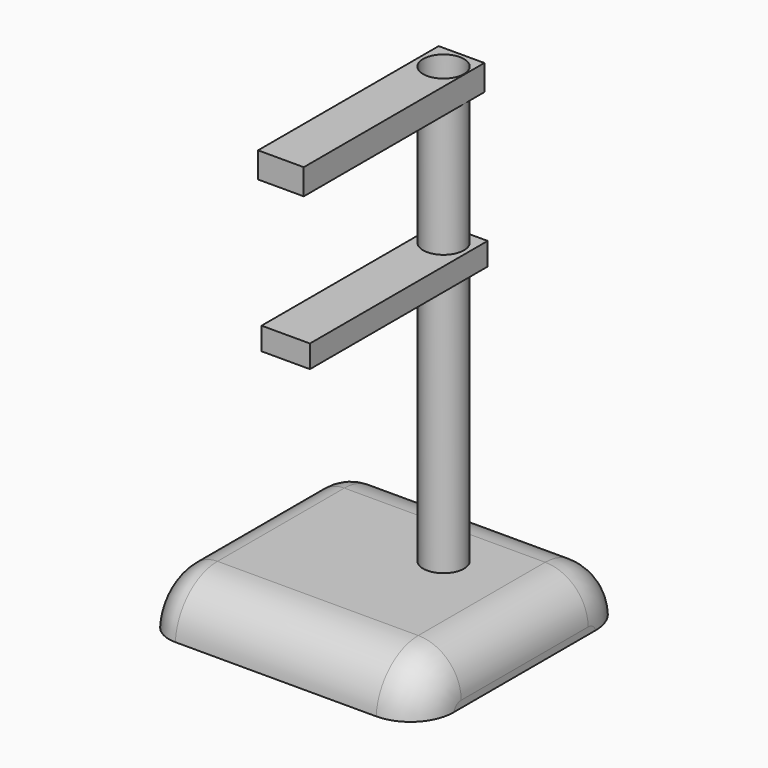
from build123d import *

# Parameters (mm, degrees)
F0_W        = 93.7904641032
F0_H        = 89.8338183761
F1_DEPTH    = 16.9549565762
F2_T1_DEPTH = 183.3558146052
F3_R        = 10.7925712466
F4_R        = 14.6181693704
F5_R        = 6.9569907431
F6_DEPTH    = 112.9271313548
F8_W        = 16.4551511407
F8_H        = 75.6539739668
F9_DEPTH    = 7.6955053955
F10_DEPTH   = 43.5431748629
F11_W       = 15.558283776
F11_H       = 76.8622979522
F11_R       = 6.9569907431
F12_DEPTH   = 8.7455324829


# Not quite as in the source:
# - a fillet or chamfer that OpenCascade refuses, or shapes differently, is made with other operations: its cross-section is extruded or revolved along the edge and cut away or added


with BuildPart() as f1:
    # F0 (on Top) → F1 (new body)
    with BuildSketch(Plane.XY):
        with Locations((8.7873749435, 5.4381676018)):
            Rectangle(F0_W, F0_H)
    extrude(amount=F1_DEPTH)

    # F2: fillet of radius 17.9401412852 on 2 edges, made by hand

    # F2_s2 → F2_t1 (cut)
    with BuildSketch(Plane.YZ.offset(-82.8905323591)):
        with BuildLine():
            ThreePointArc((-39.4787415862, 0), (-33.8980337182, 12.0440712599), (-21.5656714858, 16.9549565762))
            Line((-21.5656714858, 16.9549565762), (-39.4787415862, 16.9549565762))
            Line((-39.4787415862, 16.9549565762), (-39.4787415862, 0))
        make_face()
        with BuildLine():
            ThreePointArc((50.3550767899, 0), (44.7743689219, 12.0440712599), (32.4420066895, 16.9549565762))
            Line((32.4420066895, 16.9549565762), (50.3550767899, 16.9549565762))
            Line((50.3550767899, 16.9549565762), (50.3550767899, 0))
        make_face()
    extrude(amount=F2_T1_DEPTH, mode=Mode.SUBTRACT)

    # F3
    f3_edges = [f1.edges().sort_by_distance(p)[0] for p in [
        (-38.107857, 5.438168, 16.954957),
        (-38.107857, -33.898034, 12.044071),
        (-38.107857, 44.774369, 12.044071),
    ]]
    fillet(f3_edges, radius=F3_R)

    # F4
    f4_edges = [f1.edges().sort_by_distance(p)[0] for p in [
        (55.682607, 44.774369, 12.044071),
        (55.682607, 5.438168, 16.954957),
        (55.682607, -33.898034, 12.044071),
    ]]
    fillet(f4_edges, radius=F4_R)

    # F5 (on Top) → F6 (join)
    with BuildSketch(Plane.XY):
        with Locations((19.552404061, 16.0813909024)):
            Circle(F5_R)
    extrude(amount=F6_DEPTH)

    # F8 (on offset) → F9 (join)
    with BuildSketch(Plane.XY.offset(112.385711167)):
        with Locations((19.8183581233, -13.5854128748)):
            Rectangle(F8_W, F8_H)
    extrude(amount=-F9_DEPTH)

    # F10 (add): a face of the model
    f10_faces = [f1.faces().sort_by_distance(p)[0] for p in [
        (19.552404061, 16.0813909024, 112.9271313548),
    ]]
    extrude(f10_faces, amount=F10_DEPTH)


with BuildPart() as f12:
    # F11 (on face) → F12 (new body)
    with BuildSketch(Plane.XY.offset(156.4703062177)):
        with Locations((18.967570737, -13.9813087881)):
            Rectangle(F11_W, F11_H)
        with Locations((19.552404061, 16.0813909024)):
            Circle(F11_R, mode=Mode.SUBTRACT)
    extrude(amount=F12_DEPTH)


solid = Compound([f1.part, f12.part])
